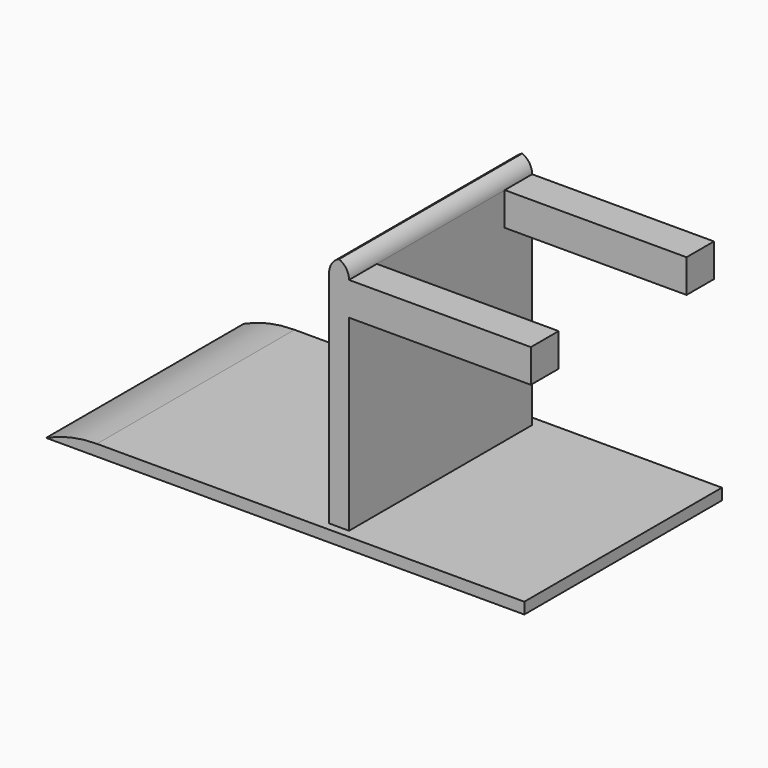
from build123d import *

# Parameters (mm, degrees)
F0_W        = 68.1868493557
F0_H        = 55.5541068316
F1_DEPTH    = 2.54
F2_T1_DEPTH = 112.6971628242
F3_W        = 4.4784088386
F3_H        = 51.4798170188
F4_DEPTH    = 53.34
F5_T1_DEPTH = 69.8761243641
F6_W        = 7.8073056648
F6_H        = 7.4690097984
F6_W_2      = 7.7111199498
F7_DEPTH    = 40.894
F8_DEPTH    = 39.37


# Not quite as in the source:
# - a fillet or chamfer that OpenCascade refuses, or shapes differently, is made with other operations: its cross-section is extruded or revolved along the edge and cut away or added


with BuildPart() as f1:
    # F0 (on Top) → F1 (new body)
    with BuildSketch(Plane.XY):
        with Locations((-34.0934246778, 27.7770534158)):
            Rectangle(F0_W, F0_H)
    extrude(amount=F1_DEPTH)

    # F2: fillet of radius 26.9812507731 on 1 edges, made by hand

    # F2_s2 → F2_t1 (cut)
    with BuildSketch(Plane.XZ.offset(-84.1256348279)):
        with BuildLine():
            ThreePointArc((-68.1868493557, 0), (-62.6119710245, 1.8973464712), (-56.7582381572, 2.54))
            Line((-56.7582381572, 2.54), (-68.1868493557, 2.54))
            Line((-68.1868493557, 2.54), (-68.1868493557, 0))
        make_face()
    extrude(amount=F2_T1_DEPTH, mode=Mode.SUBTRACT)

    # F3 (on face) → F4 (join)
    with BuildSketch(Plane.XY.offset(2.54)):
        with Locations((-3.760119027, 27.5797095965)):
            Rectangle(F3_W, F3_H)
    extrude(amount=F4_DEPTH)

    # F5: fillet of radius 3.6792614691 on 2 edges, made by hand

    # F5_s2 → F5_t1 (cut)
    with BuildSketch(Plane.XZ.offset(-62.5177717785)):
        with BuildLine():
            ThreePointArc((-1.5209146077, 52.2007385309), (-2.5985453422, 54.8023692655), (-5.2001760767, 55.88))
            Line((-5.2001760767, 55.88), (-1.5209146077, 55.88))
            Line((-1.5209146077, 55.88), (-1.5209146077, 52.2007385309))
        make_face()
        with BuildLine():
            ThreePointArc((-5.9993234463, 52.2007385309), (-4.9216927118, 54.8023692655), (-2.3200619772, 55.88))
            Line((-2.3200619772, 55.88), (-5.9993234463, 55.88))
            Line((-5.9993234463, 55.88), (-5.9993234463, 52.2007385309))
        make_face()
    extrude(amount=F5_T1_DEPTH, mode=Mode.SUBTRACT)

    # F6 (on face) → F7 (join)
    with BuildSketch(Plane.YZ.offset(-1.5209146077)):
        with Locations((5.7434539194, 48.4662336318)):
            Rectangle(F6_W, F6_H)
        with Locations((49.464058131, 48.4662336318)):
            Rectangle(F6_W_2, F6_H)
    extrude(amount=F7_DEPTH)

    # F8 (add): a face of the model
    f8_faces = [f1.faces().sort_by_distance(p)[0] for p in [
        (0, 27.7770534158, 1.27),
    ]]
    extrude(f8_faces, amount=F8_DEPTH)


solid = f1.part
